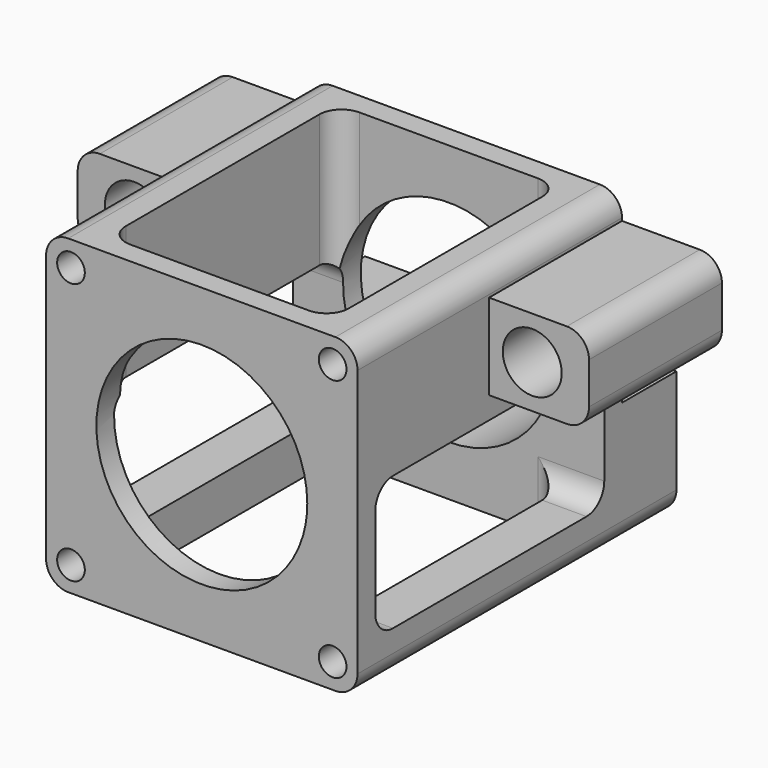
from build123d import *

# Parameters (mm, degrees)
F3_R          = 2.5
F4_DEPTH      = 42.28
F4_DEPTH_BACK = 29.68
F5_DEPTH      = 30
F5_DEPTH_BACK = 29.68
F3_W          = 18.04
F3_H          = 15.5
F3_R_2        = 5.32
F8_DEPTH      = 30
F9_START      = -20
F1_R          = 5.32
F1_R_2        = 3.41
F9_DEPTH      = 10
F10_R         = 4
F12_DEPTH     = 56.231
F14_DEPTH     = 74.271


# Not quite as in the source:
# - a feature of the source that left no trace in its solid (it failed there, or was rolled back) is left out


with BuildPart() as f4:
    # F3 (on Front) → F4 (new body, two sides)
    with BuildSketch(Plane.XZ) as f4_sk:
        with BuildLine():
            Line((-18.2932555878, -5.28), (-28.115, -5.28))
            Line((-28.115, -5.28), (-28.115, -28.115))
            Line((-28.115, -28.115), (28.115, -28.115))
            Line((28.115, -28.115), (28.115, -5.28))
            Line((28.115, -5.28), (18.2932555878, -5.28))
            ThreePointArc((18.2932555878, -5.28), (0, -19.04), (-18.2932555878, -5.28))
        make_face()
        with Locations((-23.62, -23.62)):
            Circle(F3_R, mode=Mode.SUBTRACT)
        with Locations((23.62, -23.62)):
            Circle(F3_R, mode=Mode.SUBTRACT)
    extrude(amount=-F4_DEPTH)
    extrude(f4_sk.sketch, amount=F4_DEPTH_BACK)

    # F3 (on Front) → F5 (join, two sides)
    with BuildSketch(Plane.XZ) as f5_sk:
        with BuildLine():
            Line((28.115, 28.115), (-28.115, 28.115))
            Line((-28.115, 28.115), (-28.115, 23.62))
            Line((-28.115, 23.62), (-28.115, 8.12))
            Line((-28.115, 8.12), (-28.115, -5.28))
            Line((-28.115, -5.28), (-18.2932555878, -5.28))
            ThreePointArc((-18.2932555878, -5.28), (-2.6662720799, 18.8523895885), (19.04, 0))
            ThreePointArc((19.04, 0), (18.8523895885, -2.6662720799), (18.2932555878, -5.28))
            Line((18.2932555878, -5.28), (28.115, -5.28))
            Line((28.115, -5.28), (28.115, 8.12))
            Line((28.115, 8.12), (28.115, 23.62))
            Line((28.115, 23.62), (28.115, 28.115))
        make_face()
        with Locations((-23.62, 23.62)):
            Circle(F3_R, mode=Mode.SUBTRACT)
        with Locations((23.62, 23.62)):
            Circle(F3_R, mode=Mode.SUBTRACT)
    extrude(amount=-F5_DEPTH)
    extrude(f5_sk.sketch, amount=F5_DEPTH_BACK)

    # F3 (on Front) → F8 (join)
    with BuildSketch(Plane.XZ):
        with Locations((37.135, 15.87)):
            Rectangle(F3_W, F3_H)
        with Locations((35.915, 15.87)):
            Circle(F3_R_2, mode=Mode.SUBTRACT)
        with Locations((-37.135, 15.87)):
            Rectangle(F3_W, F3_H)
        with Locations((-35.915, 15.87)):
            Circle(F3_R_2, mode=Mode.SUBTRACT)
    extrude(amount=-F8_DEPTH)

    # F1 (on Front) → F9 (join)
    with BuildSketch(Plane.XZ.offset(F9_START)):
        with Locations((35.915, 15.87)):
            Circle(F1_R)
        with Locations((35.915, 15.87)):
            Circle(F1_R_2, mode=Mode.SUBTRACT)
        with Locations((-35.915, 15.87)):
            Circle(F1_R)
        with Locations((-35.915, 15.87)):
            Circle(F1_R_2, mode=Mode.SUBTRACT)
    extrude(amount=-F9_DEPTH)

    # F10
    f10_edges = [f4.edges().sort_by_distance(p)[0] for p in [
        (-46.155, 15, 23.62),
        (-46.155, 15, 8.12),
        (-28.115, 6.3, -28.115),
        (28.115, 6.3, -28.115),
        (46.155, 15, 8.12),
        (46.155, 15, 23.62),
        (28.115, 0.16, 28.115),
        (-28.115, 0.16, 28.115),
    ]]
    fillet(f10_edges, radius=F10_R)

    # F11 (on face) → F12 (cut, through all)
    with BuildSketch(Plane.XY.offset(28.115)):
        with BuildLine():
            Line((16.115, 26), (-16.115, 26))
            ThreePointArc((-16.115, 26), (-18.9434271247, 24.8284271247), (-20.115, 22))
            Line((-20.115, 22), (-20.115, -21.68))
            ThreePointArc((-20.115, -21.68), (-18.9434271247, -24.5084271247), (-16.115, -25.68))
            Line((-16.115, -25.68), (16.115, -25.68))
            ThreePointArc((16.115, -25.68), (18.9434271247, -24.5084271247), (20.115, -21.68))
            Line((20.115, -21.68), (20.115, 22))
            ThreePointArc((20.115, 22), (18.9434271247, 24.8284271247), (16.115, 26))
        make_face()
    extrude(amount=-F12_DEPTH, mode=Mode.SUBTRACT)

    # F13 (on face) → F14 (cut, through all)
    with BuildSketch(Plane.YZ.offset(28.115)):
        with BuildLine():
            Line((22, 4.12), (-21.68, 4.12))
            ThreePointArc((-21.68, 4.12), (-24.5084271247, 2.9484271247), (-25.68, 0.12))
            Line((-25.68, 0.12), (-25.68, -16.115))
            ThreePointArc((-25.68, -16.115), (-24.5084271247, -18.9434271247), (-21.68, -20.115))
            Line((-21.68, -20.115), (22, -20.115))
            ThreePointArc((22, -20.115), (24.8284271247, -18.9434271247), (26, -16.115))
            Line((26, -16.115), (26, 0.12))
            ThreePointArc((26, 0.12), (24.8284271247, 2.9484271247), (22, 4.12))
        make_face()
    extrude(amount=-F14_DEPTH, mode=Mode.SUBTRACT)


solid = f4.part
